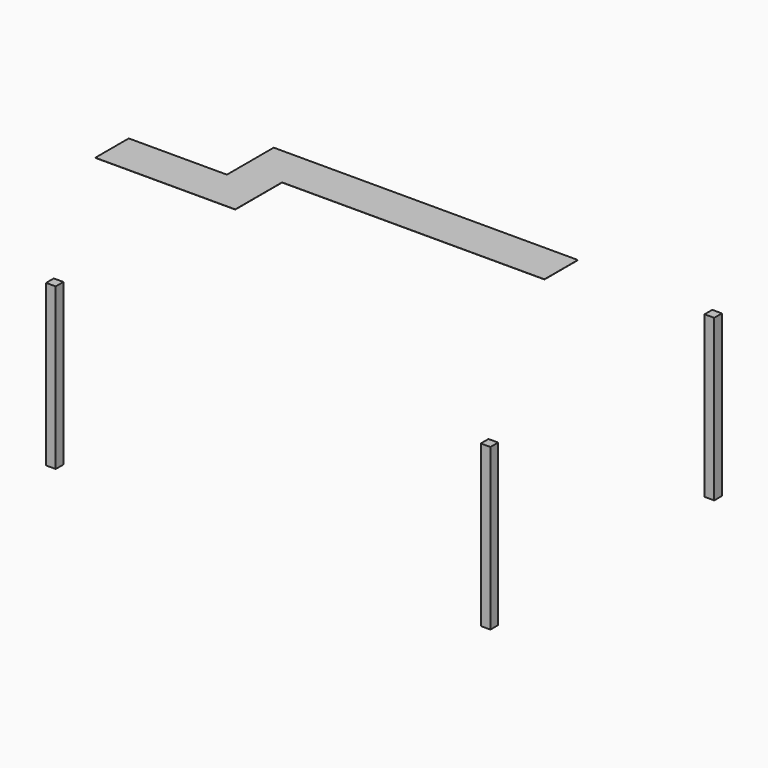
from build123d import *

# Parameters (mm, degrees)
F4_DEPTH  = 25
F7_W      = 1500
F7_H      = 1500
F11_DEPTH = 25000


# Not quite as in the source:
# - the program builds the solid bodies; features that only make, move or delete a surface that nothing else refers to are left out


with BuildPart() as f4:
    # F3 (on offset) → F4 (new body)
    with BuildSketch(Plane.XY.offset(25000)):
        Polygon((-84963.8977050781, 35900), (-84963.8977050781, 29400), (-63200, 29400), (-63200, 38500), (-22400, 38500), (-22400, 45000), (-69700, 45000), (-69700, 35900), align=None)
    extrude(amount=F4_DEPTH)


with BuildPart() as f11:
    # F7 (on Top) → F11 (new body)
    with BuildSketch(Plane.XY):
        with Locations((-750, 44250)):
            Rectangle(F7_W, F7_H)
    extrude(amount=F11_DEPTH)


with BuildPart() as f11b:
    # F7 (on Top) → F11, piece 2 (new body)
    with BuildSketch(Plane.XY):
        with Locations((-750, 750)):
            Rectangle(F7_W, F7_H)
    extrude(amount=F11_DEPTH)


with BuildPart() as f11c:
    # F7 (on Top) → F11, piece 3 (new body)
    with BuildSketch(Plane.XY):
        with Locations((-68350, 750)):
            Rectangle(F7_W, F7_H)
    extrude(amount=F11_DEPTH)


solid = Compound([f4.part, f11.part, f11b.part, f11c.part])
